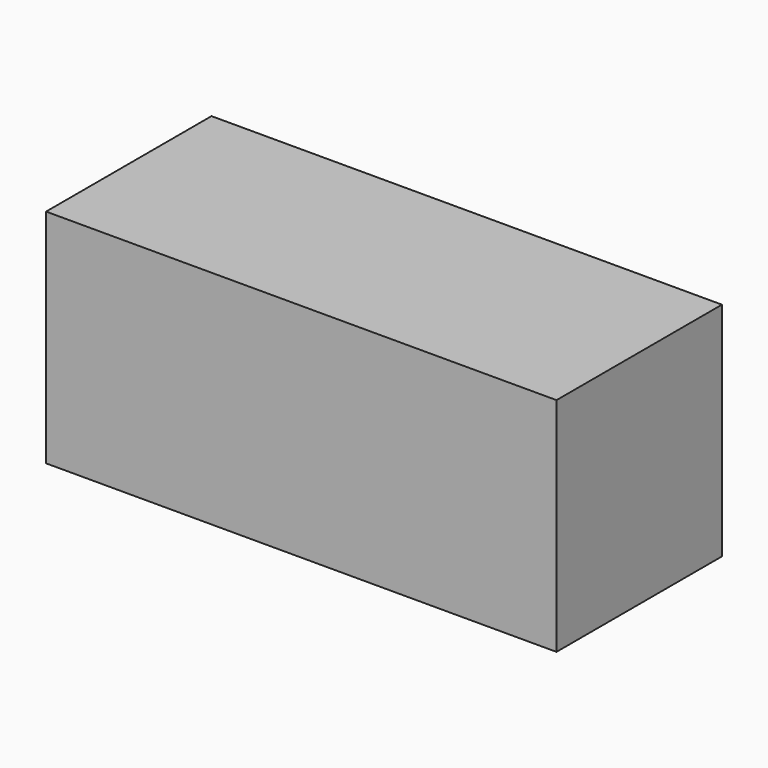
from build123d import *

# Parameters (mm, degrees)
F0_W         = 57.5743503869
F0_H         = 23.3224909753
F1_DEPTH     = 25
F2_TEXT_SIZE = 6.7766419508
F3_DEPTH     = 2


# Not quite as in the source:
# - Text() gives the source's letters only with a copy of the font that has no kerning and outlines rounded to 1/6400 em; it was checked with that copy


with BuildPart() as f1:
    # F0 (on Top) → F1 (new body)
    with BuildSketch(Plane.XY):
        with Locations((28.7871751934, -11.6612454876)):
            Rectangle(F0_W, F0_H)
    extrude(amount=F1_DEPTH)

    # F2 (on face) → F3 (join)
    with BuildSketch(Plane.XZ.offset(23.3224909753)):
        with Locations((3.3178438898, 10.2462833747)):
            Text('ADVO RODEIRA', F2_TEXT_SIZE, font='Open Sans', text_align=(TextAlign.LEFT, TextAlign.BOTTOM))
    extrude(amount=-F3_DEPTH)


solid = f1.part
